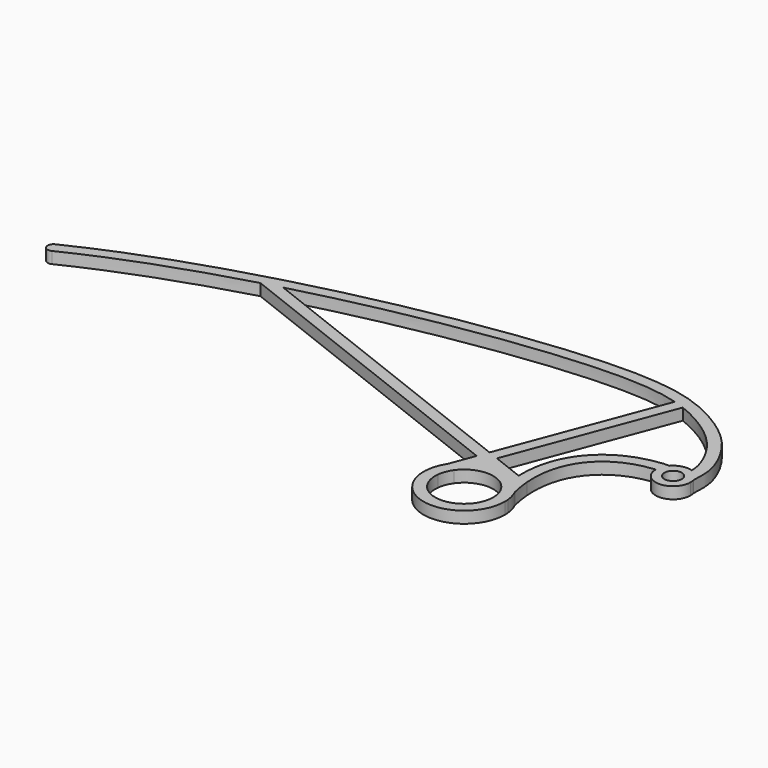
from build123d import *

# Parameters (mm, degrees)
F0_R     = 1.5
F1_DEPTH = 2


# Not quite as in the source:
# - ends of sketch curves that miss each other by under 0.0002 mm in the source are joined
# - the dataset's text gives a spline's control points without its knots; the knots are read off the source's solid
# - a feature names something its author has since deleted; it is built from what else it names


with BuildPart() as f1:
    # F0 (on Top) → F1 (new body)
    with BuildSketch(Plane.XY):
        with BuildLine():
            ThreePointArc((52.2935542038, -40.6999699993), (55.2960408024, -43.6949874982), (58.293550068, -40.6949885322))
            ThreePointArc((58.293550068, -40.6949885322), (58.2683262446, -40.3067789254), (58.1930789354, -39.9250974055))
            ThreePointArc((58.1930789354, -39.9250974055), (57.4796767246, -38.6405177387), (56.2418257324, -37.8488027926))
            ThreePointArc((56.2418257324, -37.8488027926), (54.5142276657, -37.797980318), (53.0452934588, -38.7086999783))
            ThreePointArc((53.0452934588, -38.7086999783), (52.4868923439, -39.6354261603), (52.2935542038, -40.6999699993))
        make_face()
        with Locations((55.293550068, -40.6949885322)):
            Circle(F0_R, mode=Mode.SUBTRACT)
        with BuildLine():
            ThreePointArc((56.2418257324, -37.8488027926), (57.4796767246, -38.6405177387), (58.1930789354, -39.9250974055))
            add(Edge.make_bspline(
                [(58.1930789354, -39.9250974055), (58.3033130736, -37.7310082657), (58.2243494159, -35.5108400169), (55.0379759914, -28.7548025201), (48.9442417419, -24.2694887803), (44.3900033027, -22.3203597806), (42.6738912189, -21.8107824439)],
                knots=[0, 0, 0, 0, 0.1015612411, 0.2235800295, 0.3685390699, 0.4388199083, 0.4388199083, 0.4388199083, 0.4388199083], degree=3))
            Line((42.6738912189, -21.8107824439), (41.964733286, -23.686983414))
            add(Edge.make_bspline(
                [(43.8609833986, -24.3268333981), (43.3289424335, -24.1211020721), (42.7047021585, -23.9054209924), (42.0415249398, -23.7092758985), (41.964733286, -23.686983414)],
                knots=[0.4114771922, 0.4114771922, 0.4114771922, 0.4114771922, 0.4375, 0.4408809882, 0.4408809882, 0.4408809882, 0.4408809882], degree=3))
            add(Edge.make_bspline(
                [(56.2418257324, -37.8488027926), (56.2394213733, -37.7603227769), (56.2286503864, -37.4873658698), (56.1800365415, -36.9201590877), (56.069742607, -36.3538850938), (55.8543969217, -35.6321786342), (55.5678897973, -34.8258093362), (55.0817648726, -33.7070238451), (54.3034301535, -32.2914370705), (53.5048198591, -31.1313333662), (52.7839346376, -30.2592295206), (51.9942866252, -29.4080883353), (50.8900875481, -28.3917840446), (49.39835744, -27.2551920717), (48.0378091306, -26.3838599758), (46.892639081, -25.7358249791), (45.7132806304, -25.1200272482), (44.7078870744, -24.6607216085), (43.9678542796, -24.368158577), (43.8609833986, -24.3268333981)],
                knots=[0.0398594843, 0.0398594843, 0.0398594843, 0.0398594843, 0.046875, 0.0625, 0.09375, 0.109375, 0.125, 0.15625, 0.1875, 0.21875, 0.234375, 0.25, 0.28125, 0.3125, 0.34375, 0.359375, 0.375, 0.40625, 0.4114771922, 0.4114771922, 0.4114771922, 0.4114771922], degree=3))
        make_face()
        with BuildLine():
            add(Edge.make_bspline(
                [(52.2935542038, -40.6999699993), (45.456263492, -41.3409080355), (40.3978308424, -46.0921366862), (41.0869357168, -54.4406835786)],
                knots=[0, 0, 0, 0, 18.0622051912, 18.0622051912, 18.0622051912, 18.0622051912], degree=3))
            ThreePointArc((52.2935542038, -40.6999699993), (52.4868923439, -39.6354261603), (53.0452934588, -38.7086999783))
            add(Edge.make_bspline(
                [(52.1068895218, -38.7086999783), (52.4196908341, -38.7086999783), (52.7324921465, -38.7086999783), (53.0452934588, -38.7086999783)],
                knots=[0, 0, 0, 0, 0.938403937, 0.938403937, 0.938403937, 0.938403937], degree=3))
            add(Edge.make_bspline(
                [(52.1068895218, -38.7086999783), (50.9542029326, -38.8167545733), (48.7166922252, -39.2432467553), (45.656251664, -40.5314133508), (43.0085385627, -42.4829452683), (40.9177950005, -45.0828169643), (39.5222111221, -48.2640140254), (39.0301599925, -51.2150541571), (39.0166820966, -53.0841597893), (39.0364706431, -53.640353514)],
                knots=[0, 0, 0, 0, 0.125, 0.25, 0.375, 0.5, 0.625, 0.75, 0.8013710099, 0.8013710099, 0.8013710099, 0.8013710099], degree=3))
            Line((39.0364706431, -53.640353514), (41.0869357168, -54.4406835786))
        make_face()
        with BuildLine():
            Line((41.964733286, -23.686983414), (42.6738912189, -21.8107824439))
            add(Edge.make_bspline(
                [(42.6738912189, -21.8107824439), (39.5726178708, -20.8898993454), (22.5646670262, -18.6515577464), (-27.2658854571, -27.8972020005), (-51.8069210646, -39.9311738866)],
                knots=[0.4388199083, 0.4388199083, 0.4388199083, 0.4388199083, 0.5658279827, 1, 1, 1, 1], degree=3))
            ThreePointArc((-51.8069210646, -39.9311738866), (-52.2645064284, -41.2693127564), (-50.9263675587, -41.7268981202))
            add(Edge.make_bspline(
                [(-23.2001931383, -31.4948417187), (-24.5902934046, -31.8889224129), (-30.2586462024, -33.5514164099), (-39.9245924887, -36.8107053488), (-47.460158402, -40.0272036082), (-50.9263675587, -41.7268981202)],
                knots=[0.8548139109, 0.8548139109, 0.8548139109, 0.8548139109, 0.875, 0.9375, 1, 1, 1, 1], degree=3))
            add(Edge.make_bspline(
                [(-19.9786029715, -30.6053536552), (-21.0551466867, -30.8947880406), (-22.1295355043, -31.1913200851), (-23.2001931383, -31.4948417187)],
                knots=[0.8392665501, 0.8392665501, 0.8392665501, 0.8392665501, 0.8548139109, 0.8548139109, 0.8548139109, 0.8548139109], degree=3))
            add(Edge.make_bspline(
                [(41.964733286, -23.686983414), (41.3317504553, -23.503229591), (39.9116827451, -23.1510783719), (37.4071483832, -22.746096553), (34.3488873951, -22.4920963849), (30.7487168375, -22.424981715), (26.5130652723, -22.5659356176), (20.1107293403, -23.0314333909), (10.9126678715, -24.1239147624), (-1.4091965396, -26.2175832368), (-11.9228386138, -28.5154051855), (-18.1252105086, -30.1070594376), (-19.9786029715, -30.6053536552)],
                knots=[0.4408809882, 0.4408809882, 0.4408809882, 0.4408809882, 0.46875, 0.5, 0.53125, 0.5625, 0.59375, 0.625, 0.6875, 0.75, 0.8125, 0.8392665501, 0.8392665501, 0.8392665501, 0.8392665501], degree=3))
        make_face()
        with BuildLine():
            add(Edge.make_bspline(
                [(41.0869357168, -54.4406835786), (41.171365149, -55.4635512139), (41.3420723504, -56.5404191219), (41.6063564607, -57.670343851)],
                knots=[18.0622051912, 18.0622051912, 18.0622051912, 18.0622051912, 20.2751945115, 20.2751945115, 20.2751945115, 20.2751945115], degree=3))
            Line((41.0869357168, -54.4406835786), (39.0364758665, -53.6403401319))
            Line((39.0364758665, -53.6403401319), (33.5854085722, -51.5126583899))
            Line((33.5854085722, -51.5126583899), (32.8782428587, -53.383588596))
            Line((32.8782428587, -53.383588596), (33.9898275109, -53.8174666315))
            ThreePointArc((33.9898275109, -53.8174666315), (38.453280426, -54.4487013098), (41.6063564607, -57.670343851))
        make_face()
        with BuildLine():
            Line((33.5854085722, -51.5126583899), (43.8609833986, -24.3268333981))
            add(Edge.make_bspline(
                [(43.8609833986, -24.3268333981), (43.3289424335, -24.1211020721), (42.7047021585, -23.9054209924), (42.0415249398, -23.7092758985), (41.964733286, -23.686983414)],
                knots=[0.4114771922, 0.4114771922, 0.4114771922, 0.4114771922, 0.4375, 0.4408809882, 0.4408809882, 0.4408809882, 0.4408809882], degree=3))
            Line((41.964733286, -23.686983414), (31.7221959356, -50.7854020024))
            Line((31.7221959356, -50.7854020024), (33.5854085722, -51.5126583899))
        make_face()
        with BuildLine():
            ThreePointArc((42.257771215, -59.9881478041), (42.032460875, -58.8010294155), (41.6063564607, -57.670343851))
            add(Edge.make_bspline(
                [(41.6063564607, -57.670343851), (41.7816276486, -58.4197012349), (41.9980562098, -59.1923942837), (42.257771215, -59.9881478041)],
                knots=[20.2751945115, 20.2751945115, 20.2751945115, 20.2751945115, 21.7428319964, 21.7428319964, 21.7428319964, 21.7428319964], degree=3))
        make_face()
        with BuildLine():
            add(Edge.make_bspline(
                [(41.6063564607, -57.670343851), (41.7816276486, -58.4197012349), (41.9980562098, -59.1923942837), (42.257771215, -59.9881478041)],
                knots=[20.2751945115, 20.2751945115, 20.2751945115, 20.2751945115, 21.7428319964, 21.7428319964, 21.7428319964, 21.7428319964], degree=3))
            ThreePointArc((41.6063564607, -57.670343851), (38.453280426, -54.4487013098), (33.9898275109, -53.8174666315))
            ThreePointArc((33.9898275109, -53.8174666315), (33.2574115394, -53.9976651943), (32.5486357461, -54.2556216871))
            ThreePointArc((32.5486357461, -54.2556216871), (30.7811233168, -55.3435396802), (29.4103052988, -56.9019118146))
            Line((29.4103052988, -56.9019118146), (28.3722521988, -59.6482622997))
            ThreePointArc((28.3722521988, -59.6482622997), (34.7687096562, -67.6752852696), (42.293550068, -60.6949885322))
            ThreePointArc((42.293550068, -60.6949885322), (42.2845996326, -60.3411156944), (42.257771215, -59.9881478041))
        make_face()
        with BuildLine():
            ThreePointArc((31.1997706158, -57.824279596), (36.7987249314, -55.9269230303), (40.293550068, -60.6949885322))
            ThreePointArc((40.293550068, -60.6949885322), (35.0156984919, -65.6872624131), (30.3244306673, -60.1401440657))
            ThreePointArc((30.3244306673, -60.1401440657), (30.6164953361, -58.9271765979), (31.1997706158, -57.824279596))
        make_face(mode=Mode.SUBTRACT)
        Polygon((32.8782428587, -53.383588596), (33.5854085722, -51.5126583899), (31.7221959356, -50.7854020024), (31.015030222, -52.6563322085), align=None)
        with BuildLine():
            Line((31.015030222, -52.6563322085), (31.7221959356, -50.7854020024))
            Line((31.7221959356, -50.7854020024), (-19.9786054149, -30.6053445671))
            add(Edge.make_bspline(
                [(-19.9786054149, -30.6053445671), (-21.0551466867, -30.8947880406), (-22.1295355043, -31.1913200851), (-23.2001931383, -31.4948417187)],
                knots=[0.8392665501, 0.8392665501, 0.8392665501, 0.8392665501, 0.8548139109, 0.8548139109, 0.8548139109, 0.8548139109], degree=3))
            Line((-23.2001931383, -31.4948417187), (31.015030222, -52.6563322085))
        make_face()
        with BuildLine():
            ThreePointArc((32.5486357461, -54.2556216871), (33.2574115394, -53.9976651943), (33.9898275109, -53.8174666315))
            Line((33.9898275109, -53.8174666315), (32.8782428587, -53.383588596))
            Line((32.8782428587, -53.383588596), (32.5486357461, -54.2556216871))
        make_face()
        with BuildLine():
            Line((32.5486357461, -54.2556216871), (32.8782428587, -53.383588596))
            Line((32.8782428587, -53.383588596), (31.015030222, -52.6563322085))
            Line((31.015030222, -52.6563322085), (29.4103052988, -56.9019118146))
            ThreePointArc((29.4103052988, -56.9019118146), (30.7811233168, -55.3435396802), (32.5486357461, -54.2556216871))
        make_face()
        with BuildLine():
            Line((28.3722521988, -59.6482622997), (29.4103052988, -56.9019118146))
            ThreePointArc((29.4103052988, -56.9019118146), (28.7456734434, -58.2200518242), (28.3722521988, -59.6482622997))
        make_face()
    extrude(amount=F1_DEPTH)


solid = f1.part
